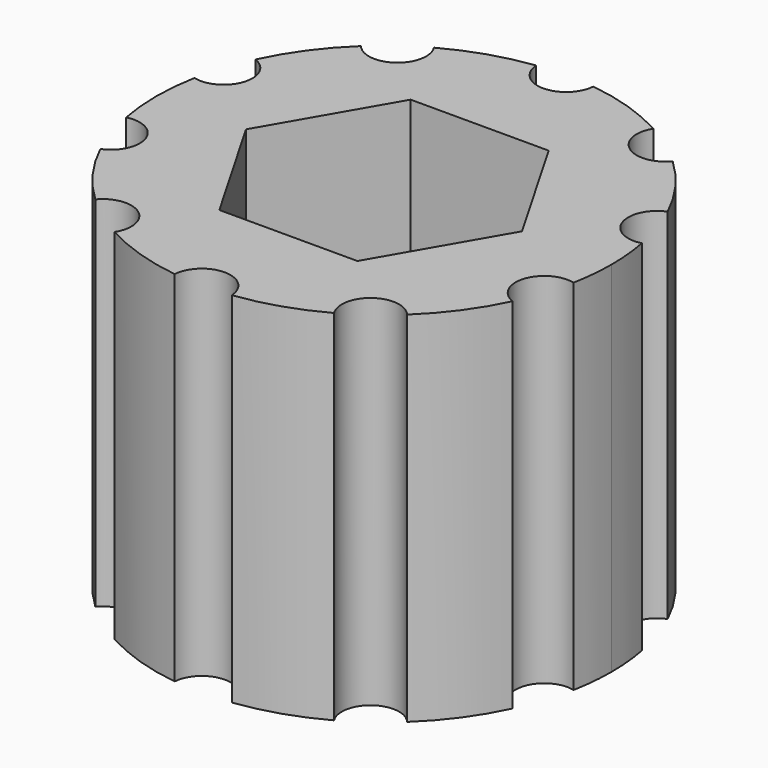
from build123d import *

# Parameters (mm, degrees)
F1_DEPTH = 15
F2_R     = 3
F3_DEPTH = 15.001
F4_R     = 3
F5_DEPTH = 10


with BuildPart() as f1:
    # F0 (on Top) → F1 (new body)
    with BuildSketch(Plane.XY):
        with BuildLine():
            ThreePointArc((9.3561974046, -1.7852717232), (9.4827054494, -0.8966171761), (9.525, 0))
            ThreePointArc((9.525, 0), (9.4827054494, 0.8966171761), (9.3561974046, 1.7852717232))
            ThreePointArc((9.3561974046, 1.7852717232), (7.9216471704, 2.5738991923), (8.6186790933, 4.0551196883))
            ThreePointArc((8.6186790933, 4.0551196883), (7.7058868714, 5.5986545281), (6.5199663128, 6.9437500156))
            ThreePointArc((6.5199663128, 6.9437500156), (4.8958471982, 6.738555569), (4.5891183065, 8.3465932074))
            ThreePointArc((4.5891183065, 8.3465932074), (2.9433868714, 9.0588133177), (1.193329695, 9.4499518115))
            ThreePointArc((1.193329695, 9.4499518115), (0, 8.3293127534), (-1.193329695, 9.4499518115))
            ThreePointArc((-1.193329695, 9.4499518115), (-2.9433868714, 9.0588133177), (-4.5891183065, 8.3465932074))
            ThreePointArc((-4.5891183065, 8.3465932074), (-4.4504477573, 8.039487236), (-4.4029672815, 7.7058868714))
            ThreePointArc((-4.4029672815, 7.7058868714), (-5.1936438859, 6.5808827064), (-6.5199663128, 6.9437500156))
            ThreePointArc((-6.5199663128, 6.9437500156), (-7.7058868714, 5.5986545281), (-8.6186790933, 4.0551196883))
            ThreePointArc((-8.6186790933, 4.0551196883), (-8.0698919683, 3.6154750772), (-7.8631260711, 2.9433868714))
            ThreePointArc((-7.8631260711, 2.9433868714), (-8.3259799016, 1.9985995007), (-9.3561974046, 1.7852717232))
            ThreePointArc((-9.3561974046, 1.7852717232), (-9.525, 0), (-9.3561974046, -1.7852717232))
            ThreePointArc((-9.3561974046, -1.7852717232), (-8.3259799016, -1.9985995007), (-7.8631260711, -2.9433868714))
            ThreePointArc((-7.8631260711, -2.9433868714), (-8.0698919683, -3.6154750772), (-8.6186790933, -4.0551196883))
            ThreePointArc((-8.6186790933, -4.0551196883), (-7.7058868714, -5.5986545281), (-6.5199663128, -6.9437500156))
            ThreePointArc((-6.5199663128, -6.9437500156), (-5.1936438859, -6.5808827064), (-4.4029672815, -7.7058868714))
            ThreePointArc((-4.4029672815, -7.7058868714), (-4.4504477573, -8.039487236), (-4.5891183065, -8.3465932074))
            ThreePointArc((-4.5891183065, -8.3465932074), (-2.9433868714, -9.0588133177), (-1.193329695, -9.4499518115))
            ThreePointArc((-1.193329695, -9.4499518115), (0, -8.3293127534), (1.193329695, -9.4499518115))
            ThreePointArc((1.193329695, -9.4499518115), (2.9433868714, -9.0588133177), (4.5891183065, -8.3465932074))
            ThreePointArc((4.5891183065, -8.3465932074), (4.8958471982, -6.738555569), (6.5199663128, -6.9437500156))
            ThreePointArc((6.5199663128, -6.9437500156), (7.7058868714, -5.5986545281), (8.6186790933, -4.0551196883))
            ThreePointArc((8.6186790933, -4.0551196883), (7.9216471704, -2.5738991923), (9.3561974046, -1.7852717232))
        make_face()
    extrude(amount=F1_DEPTH)

    # F2 (on face) → F3 (cut, through all)
    with BuildSketch(Plane.XY.offset(15)):
        Circle(F2_R)
    extrude(amount=-F3_DEPTH, mode=Mode.SUBTRACT)

    # F4 (on face) → F5 (cut)
    with BuildSketch(Plane.XY.offset(15)):
        Polygon((2.8867513459, -5), (5.7735026919, 0), (2.8867513459, 5), (-2.8867513459, 5), (-5.7735026919, 0), (-2.8867513459, -5), align=None)
        Circle(F4_R, mode=Mode.SUBTRACT)
    extrude(amount=-F5_DEPTH, mode=Mode.SUBTRACT)


solid = f1.part
